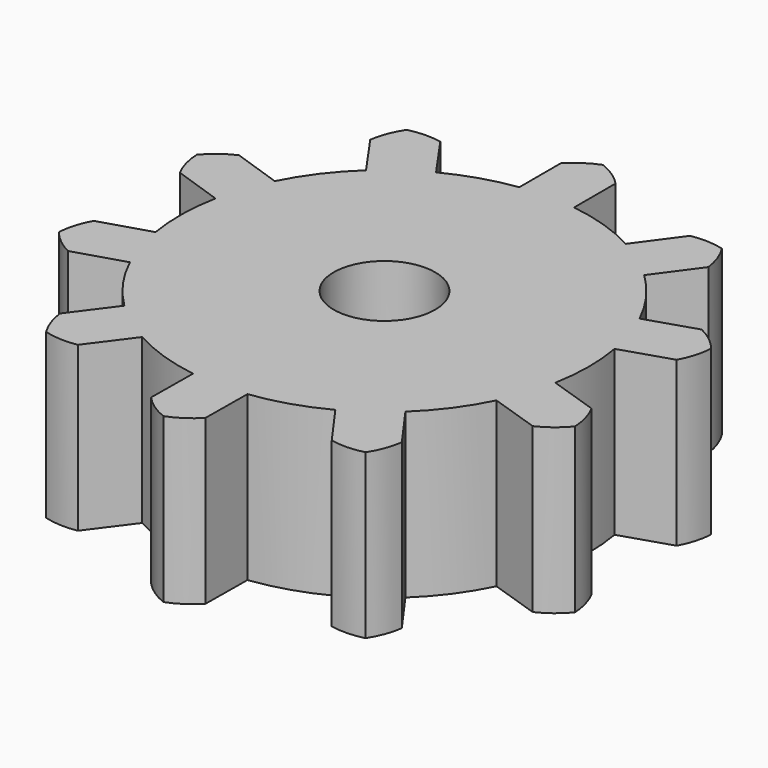
from build123d import *

# Parameters (mm, degrees)
F0_R     = 3.1
F1_DEPTH = 10


with BuildPart() as f1:
    # F0 (on Top) → F1 (new body)
    with BuildSketch(Plane.XY):
        with BuildLine():
            ThreePointArc((1.673929859, 12.3874113045), (0, 12.5), (-1.673929859, 12.3874113045))
            ThreePointArc((-1.673929859, 12.3874113045), (-3.7588224938, 11.9214618844), (-5.7339241657, 11.1073000167))
            ThreePointArc((-5.7339241657, 11.1073000167), (-7.1697054544, 10.2394005536), (-8.4763302976, 9.1870465703))
            ThreePointArc((-8.4763302976, 9.1870465703), (-9.9902333855, 7.5130045191), (-11.1784184623, 5.5940111443))
            ThreePointArc((-11.1784184623, 5.5940111443), (-11.8268519609, 4.0466742757), (-12.2622342862, 2.4264398427))
            ThreePointArc((-12.2622342862, 2.4264398427), (-12.4986778991, 0.1817987206), (-12.3276190694, -2.0687697022))
            ThreePointArc((-12.3276190694, -2.0687697022), (-11.9395449954, -3.7009816676), (-11.336389674, -5.2665234414))
            ThreePointArc((-11.336389674, -5.2665234414), (-10.2045206414, -7.2192630149), (-8.7399470524, -8.9366283084))
            ThreePointArc((-8.7399470524, -8.9366283084), (-7.4644823963, -10.0265399094), (-6.0545511265, -10.9358315027))
            ThreePointArc((-6.0545511265, -10.9358315027), (-3.9892887467, -11.8463317232), (-1.7939610174, -12.3705983634))
            ThreePointArc((-1.7939610174, -12.3705983634), (-0.1212015211, -12.4994123938), (1.5537413227, -12.4030596186))
            ThreePointArc((1.5537413227, -12.4030596186), (3.7588224938, -11.9214618844), (5.8413523551, -11.0511810529))
            ThreePointArc((5.8413523551, -11.0511810529), (7.2686508911, -10.1694008783), (8.5650105596, -9.1044271711))
            ThreePointArc((8.5650105596, -9.1044271711), (10.0626107657, -7.4157848255), (11.2321331944, -5.4853608726))
            ThreePointArc((11.2321331944, -5.4853608726), (11.8655330447, -3.9318094519), (12.285184913, -2.3074296637))
            ThreePointArc((12.285184913, -2.3074296637), (12.4998530976, -0.0606014727), (12.3069805238, 2.188202547))
            ThreePointArc((12.3069805238, 2.188202547), (11.9030985667, 3.8165749712), (11.2847919153, 5.3761948838))
            ThreePointArc((11.2847919153, 5.3761948838), (10.1340420896, 7.3178679221), (8.6528855651, 9.0209518011))
            ThreePointArc((8.6528855651, 9.0209518011), (7.3669129512, 10.0984451065), (5.9482313582, 10.9940230903))
            ThreePointArc((5.9482313582, 10.9940230903), (3.8742377423, 11.8844554741), (1.673929859, 12.3874113045))
        make_face()
        Circle(F0_R, mode=Mode.SUBTRACT)
        with BuildLine():
            ThreePointArc((-12.2622342862, 2.4264398427), (-11.8268519609, 4.0466742757), (-11.1784184623, 5.5940111443))
            Line((-11.1784184623, 5.5940111443), (-14.1805287895, 6.6212128607))
            ThreePointArc((-14.1805287895, 6.6212128607), (-15.0512360756, 6.1003265438), (-15.786995451, 5.4016765064))
            ThreePointArc((-15.786995451, 5.4016765064), (-15.6334500279, 4.3987420438), (-15.2643446134, 3.4536415591))
            Line((-15.2643446134, 3.4536415591), (-12.2622342862, 2.4264398427))
        make_face()
        with BuildLine():
            ThreePointArc((-11.336389674, -5.2665234414), (-11.9395449954, -3.7009816676), (-12.3276190694, -2.0687697022))
            Line((-12.3276190694, -2.0687697022), (-15.3583352271, -3.0082213265))
            ThreePointArc((-15.3583352271, -3.0082213265), (-15.7547724734, -3.9421866593), (-15.9374230058, -4.9402310051))
            ThreePointArc((-15.9374230058, -4.9402310051), (-15.2222949332, -5.6599848332), (-14.3671058317, -6.2059750657))
            Line((-14.3671058317, -6.2059750657), (-11.336389674, -5.2665234414))
        make_face()
        with BuildLine():
            ThreePointArc((-6.0545511265, -10.9358315027), (-7.4644823963, -10.0265399094), (-8.7399470524, -8.9366283084))
            Line((-8.7399470524, -8.9366283084), (-10.6347200455, -11.4817501301))
            ThreePointArc((-10.6347200455, -11.4817501301), (-10.4045567225, -12.4699194364), (-9.9639151672, -13.3838607655))
            ThreePointArc((-9.9639151672, -13.3838607655), (-8.9619915366, -13.5438694265), (-7.9493241196, -13.4809533245))
            Line((-7.9493241196, -13.4809533245), (-6.0545511265, -10.9358315027))
        make_face()
        with BuildLine():
            ThreePointArc((1.5537413227, -12.4030596186), (-0.1212015211, -12.4994123938), (-1.7939610174, -12.3705983634))
            Line((-1.7939610174, -12.3705983634), (-1.8247266294, -15.5434304201))
            ThreePointArc((-1.8247266294, -15.5434304201), (-1.0564027139, -16.2061008466), (-0.1617850522, -16.6847583155))
            ThreePointArc((-0.1617850522, -16.6847583155), (0.7419462008, -16.2235386762), (1.5229757107, -15.5758916753))
            Line((1.5229757107, -15.5758916753), (1.5537413227, -12.4030596186))
        make_face()
        with BuildLine():
            Line((10.4100739777, -11.6858126065), (8.5650105596, -9.1044271711))
            ThreePointArc((8.5650105596, -9.1044271711), (7.2686508911, -10.1694008783), (5.8413523551, -11.0511810529))
            Line((5.8413523551, -11.0511810529), (7.6864157733, -13.6325664882))
            ThreePointArc((7.6864157733, -13.6325664882), (8.6976727518, -13.71510773), (9.7025107722, -13.5745577889))
            ThreePointArc((9.7025107722, -13.5745577889), (10.1607920135, -12.6693329344), (10.4100739777, -11.6858126065))
        make_face()
        with BuildLine():
            Line((15.2971139884, -3.3054742658), (12.285184913, -2.3074296637))
            ThreePointArc((12.285184913, -2.3074296637), (11.8655330447, -3.9318094519), (11.2321331944, -5.4853608726))
            Line((11.2321331944, -5.4853608726), (14.2440622698, -6.4834054748))
            ThreePointArc((14.2440622698, -6.4834054748), (15.1096780482, -5.9541011602), (15.8386286408, -5.2483499528))
            ThreePointArc((15.8386286408, -5.2483499528), (15.6753658611, -4.2469514318), (15.2971139884, -3.3054742658))
        make_face()
        with BuildLine():
            Line((14.3062565663, 6.3449885386), (11.2847919153, 5.3761948838))
            ThreePointArc((11.2847919153, 5.3761948838), (11.9030985667, 3.8165749712), (12.3069805238, 2.188202547))
            Line((12.3069805238, 2.188202547), (15.3284451748, 3.1569962018))
            ThreePointArc((15.3284451748, 3.1569962018), (15.7158079437, 4.0947615341), (15.8887727305, 5.0945299651))
            ThreePointArc((15.8887727305, 5.0945299651), (15.1666994543, 5.8073159898), (14.3062565663, 6.3449885386))
        make_face()
        with BuildLine():
            Line((7.81823747, 13.5573972192), (5.9482313582, 10.9940230903))
            ThreePointArc((5.9482313582, 10.9940230903), (7.3669129512, 10.0984451065), (8.6528855651, 9.0209518011))
            Line((8.6528855651, 9.0209518011), (10.5228916769, 11.58432593))
            ThreePointArc((10.5228916769, 11.58432593), (10.2831577637, 12.5702170924), (9.833675236, 13.4798429443))
            ThreePointArc((9.833675236, 13.4798429443), (8.8302472408, 13.6301293101), (7.81823747, 13.5573972192))
        make_face()
        with BuildLine():
            Line((-1.673929859, 15.5603925183), (-1.673929859, 12.3874113045))
            ThreePointArc((-1.673929859, 12.3874113045), (0, 12.5), (1.673929859, 12.3874113045))
            Line((1.673929859, 12.3874113045), (1.673929859, 15.5603925183))
            ThreePointArc((1.673929859, 15.5603925183), (0.8992167282, 16.2155820315), (0, 16.6855426777))
            ThreePointArc((0, 16.6855426777), (-0.8992167282, 16.2155820315), (-1.673929859, 15.5603925183))
        make_face()
        with BuildLine():
            ThreePointArc((-8.4763302976, 9.1870465703), (-7.1697054544, 10.2394005536), (-5.7339241657, 11.1073000167))
            Line((-5.7339241657, 11.1073000167), (-7.5538714229, 13.7064540645))
            ThreePointArc((-7.5538714229, 13.7064540645), (-8.5642805338, 13.7987966969), (-9.5704341076, 13.6679963945))
            ThreePointArc((-9.5704341076, 13.6679963945), (-10.0374709761, 12.767257644), (-10.2962775548, 11.7862006181))
            Line((-10.2962775548, 11.7862006181), (-8.4763302976, 9.1870465703))
        make_face()
    extrude(amount=F1_DEPTH)


solid = f1.part
